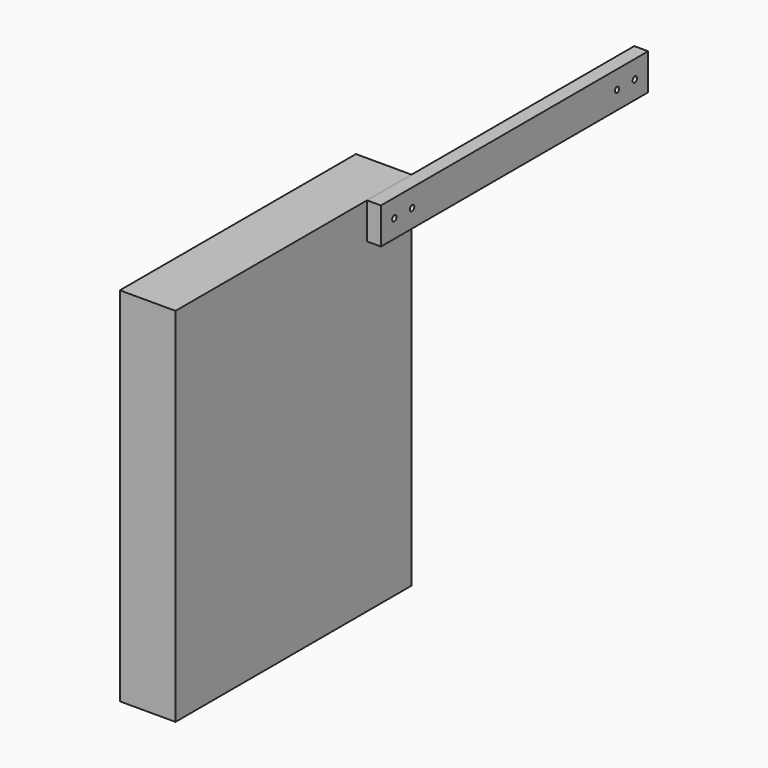
from build123d import *

# Parameters (mm, degrees)
F0_W     = 100
F0_H     = 100
F1_DEPTH = 650
F2_R     = 5
F3_DEPTH = 100.001
F4_W     = 600
F4_H     = 65
F4_R     = 5
F5_DEPTH = 25
F6_DEPTH = 430


with BuildPart() as f1:
    # F0 (on Top) → F1 (new body)
    with BuildSketch(Plane.XY):
        with Locations((-50, -50)):
            Rectangle(F0_W, F0_H)
    extrude(amount=F1_DEPTH)

    # F2 (on face) → F3 (cut, through all)
    with BuildSketch(Plane.YZ):
        with Locations((-70, 617.5)):
            Circle(F2_R)
        with Locations((-30, 617.5)):
            Circle(F2_R)
    extrude(amount=-F3_DEPTH, mode=Mode.SUBTRACT)

    # F6 (add): a face of the model
    f6_faces = [f1.faces().sort_by_distance(p)[0] for p in [
        (-50, -100, 325),
    ]]
    extrude(f6_faces, amount=F6_DEPTH)


with BuildPart() as f5:
    # F4 (on Right) → F5 (new body)
    with BuildSketch(Plane.YZ):
        with Locations((200, 617.5)):
            Rectangle(F4_W, F4_H)
        with Locations((-70, 617.5)):
            Circle(F4_R, mode=Mode.SUBTRACT)
        with Locations((-30, 617.5)):
            Circle(F4_R, mode=Mode.SUBTRACT)
        with Locations((430, 617.5)):
            Circle(F4_R, mode=Mode.SUBTRACT)
        with Locations((470, 617.5)):
            Circle(F4_R, mode=Mode.SUBTRACT)
    extrude(amount=F5_DEPTH)


solid = Compound([f1.part, f5.part])
